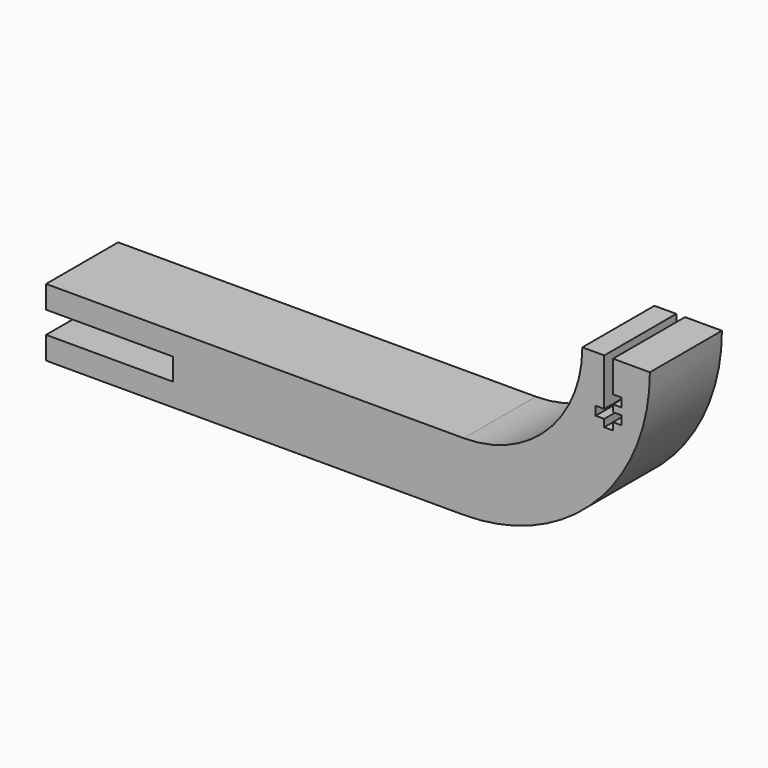
from build123d import *

# Parameters (mm, degrees)
F1_DEPTH = 11


# Not quite as in the source:
# - ends of sketch curves that miss each other by under 0.0002 mm in the source are joined
# - a feature names something its author has since deleted; it is built from what else it names


with BuildPart() as f1:
    # F0 (on Front) → F1 (new body, symmetric)
    with BuildSketch(Plane.XZ):
        Polygon((-51.0195, -8.25), (51.0195, -8.25), (51.0195, 8.25), (-51.0195, 8.25), (-51.0195, 2.7), (-20.0195, 2.7), (-20.0195, -2.7), (-51.0195, -2.7), align=None)
        with BuildLine():
            Line((51.0195, 8.25), (51.0195, -8.25))
            ThreePointArc((51.0195, -8.25), (83.1651110764, 5.0651480786), (96.4802591551, 37.2107591551))
            Line((96.4802591551, 37.2107591551), (87.4802576721, 37.2107591551))
            Line((87.4802576721, 37.2107591551), (87.4802576721, 29.5374569684))
            Line((87.4802576721, 29.5374569684), (89.5802576721, 29.5374569684))
            Line((89.5802576721, 29.5374569684), (89.5802576721, 27.3874569684))
            Line((89.5802576721, 27.3874569684), (87.4802576721, 27.3874569684))
            Line((87.4802576721, 27.3874569684), (87.4802576721, 25.7107576162))
            Line((87.4802576721, 25.7107576162), (89.5802576721, 25.7107576162))
            Line((89.5802576721, 25.7107576162), (89.5802576721, 23.5607576162))
            Line((89.5802576721, 23.5607576162), (87.4802576721, 23.5607576162))
            Line((87.4802576721, 23.5607576162), (87.4802576721, 21.7607576162))
            Line((87.4802576721, 21.7607576162), (85.3302576721, 21.7607576162))
            Line((85.3302576721, 21.7607576162), (85.3302576721, 23.5607576162))
            Line((85.3302576721, 23.5607576162), (83.2302576721, 23.5607576162))
            Line((83.2302576721, 23.5607576162), (83.2302576721, 25.7107576162))
            Line((83.2302576721, 25.7107576162), (85.3302576721, 25.7107576162))
            Line((85.3302576721, 25.7107576162), (85.3302576721, 37.2107591551))
            Line((85.3302576721, 37.2107591551), (79.9802576721, 37.2107591551))
            ThreePointArc((79.9802576721, 37.2107591551), (71.4978497843, 16.7324093708), (51.0195, 8.25))
        make_face()
    extrude(amount=F1_DEPTH, both=True)


solid = f1.part
